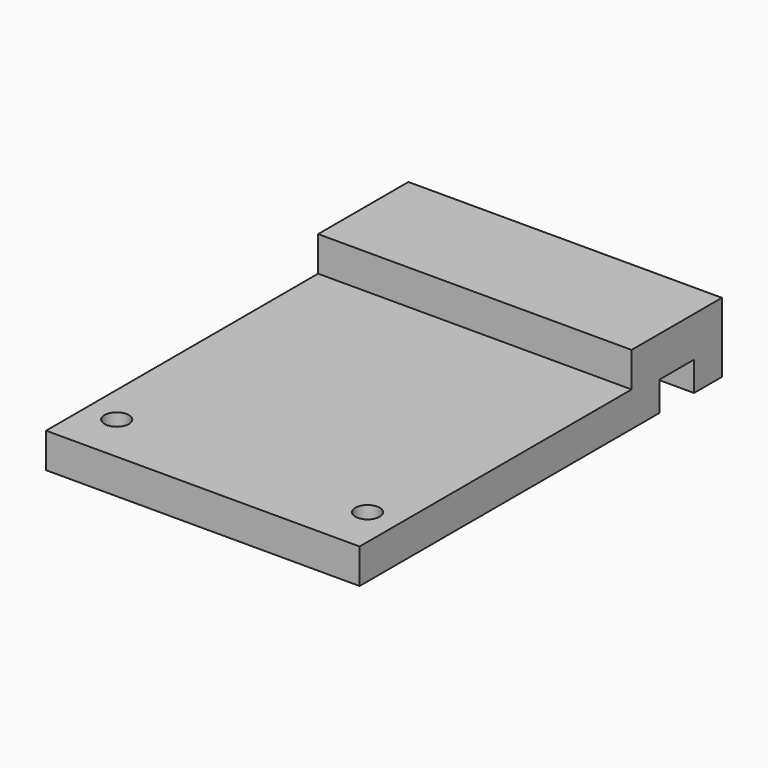
from build123d import *

# Parameters (mm, degrees)
F1_W     = 45
F1_H     = 5
F1_H_2   = 6.2
F1_H_3   = 53.8
F1_R     = 1.75
F2_DEPTH = 10
F3_DEPTH = 4.22
F4_W     = 45
F4_H     = 48.8
F4_R     = 1.75
F5_DEPTH = 5


# Not quite as in the source:
# - a feature of the source that left no trace in its solid (it failed there, or was rolled back) is left out


with BuildPart() as f2:
    # F1 (on Top) → F2 (new body)
    with BuildSketch(Plane.XY):
        with Locations((0, 30)):
            Rectangle(F1_W, F1_H)
        with Locations((0, 24.4)):
            Rectangle(F1_W, F1_H_2)
        with Locations((0, -5.6)):
            Rectangle(F1_W, F1_H_3)
        with Locations((-18, -25.45)):
            Circle(F1_R, mode=Mode.SUBTRACT)
        with Locations((18, -25.45)):
            Circle(F1_R, mode=Mode.SUBTRACT)
    extrude(amount=F2_DEPTH)

    # F1 (on Top) → F3 (cut)
    with BuildSketch(Plane.XY):
        with Locations((0, 24.4)):
            Rectangle(F1_W, F1_H_2)
    extrude(amount=F3_DEPTH, mode=Mode.SUBTRACT)

    # F4 (on face) → F5 (cut)
    with BuildSketch(Plane.XY.offset(10)):
        with Locations((0, -8.1)):
            Rectangle(F4_W, F4_H)
        with Locations((-18, -25.45)):
            Circle(F4_R, mode=Mode.SUBTRACT)
        with Locations((18, -25.45)):
            Circle(F4_R, mode=Mode.SUBTRACT)
    extrude(amount=-F5_DEPTH, mode=Mode.SUBTRACT)


solid = f2.part
